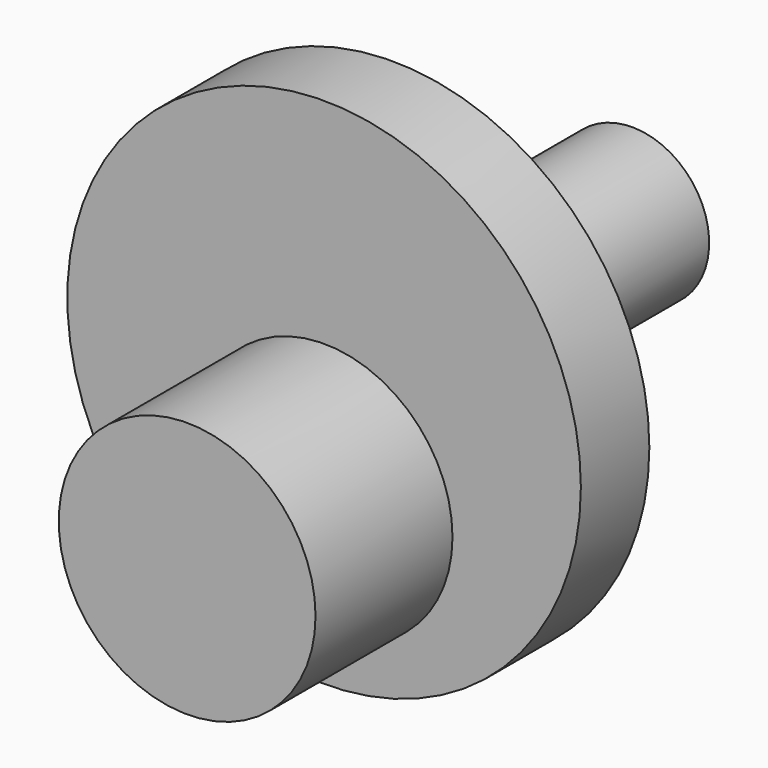
from build123d import *

# Parameters (mm, degrees)
F0_R     = 76.2
F1_DEPTH = 25.4
F2_R     = 38.1
F3_DEPTH = 76.2
F5_R     = 43.7488165657
F6_DEPTH = 25.4
F7_R     = 22.8249074769
F8_DEPTH = 63.5


# Not quite as in the source:
# - the program builds the solid bodies; features that only make, move or delete a surface that nothing else refers to are left out


with BuildPart() as f1:
    # F0 (on Front) → F1 (new body)
    with BuildSketch(Plane.XZ):
        Circle(F0_R)
    extrude(amount=F1_DEPTH)


with BuildPart() as f3:
    # F2 (on Front) → F3 (new body)
    with BuildSketch(Plane.XZ):
        with Locations((0, -25.4)):
            Circle(F2_R)
    extrude(amount=F3_DEPTH)


with BuildPart() as f6:
    # F5 (on face) → F6 (new body)
    with BuildSketch(Plane(origin=(0, 0, 0), x_dir=(-1, 0, 0), z_dir=(0, 1, 0))):
        Circle(F5_R)
    extrude(amount=F6_DEPTH)


with BuildPart() as f8:
    # F7 (on face) → F8 (new body)
    with BuildSketch(Plane(origin=(0, 25.4, 0), x_dir=(-1, 0, 0), z_dir=(0, 1, 0))):
        Circle(F7_R)
    extrude(amount=F8_DEPTH)


solid = Compound([f1.part, f3.part, f6.part, f8.part])
